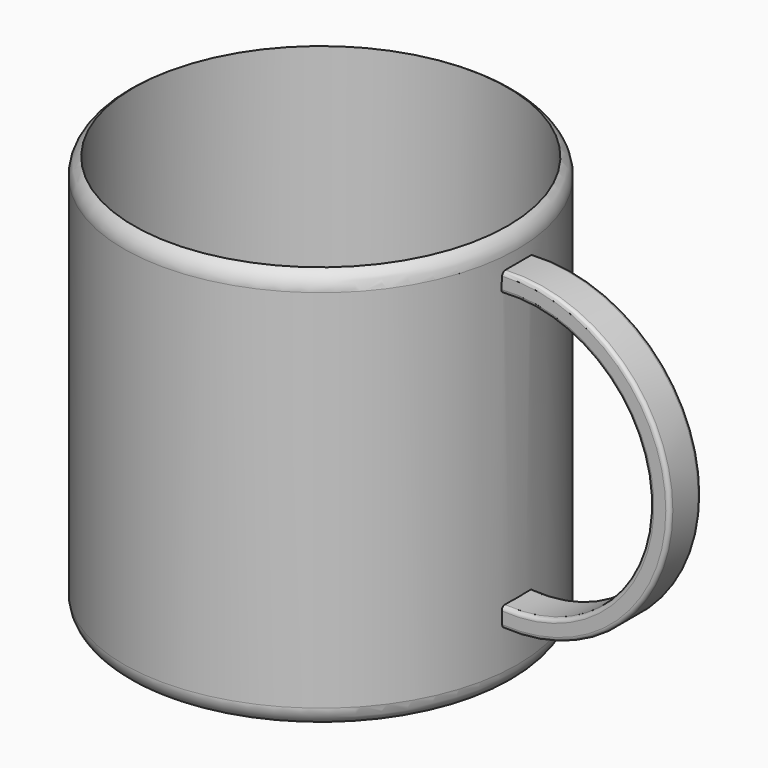
from build123d import *

# Parameters (mm, degrees)
F0_R     = 50
F0_R_2   = 47.5
F1_DEPTH = 101.6
F4_DEPTH = 5
F6_DEPTH = 5
F7_F1_R  = 1
F7_F2_R  = 1
F7_F3_R  = 1
F7_F4_R  = 1


# Not quite as in the source:
# - a fillet or chamfer that OpenCascade refuses, or shapes differently, is made with other operations: its cross-section is extruded or revolved along the edge and cut away or added


with BuildPart() as f1:
    # F0 (on Top) → F1 (new body)
    with BuildSketch(Plane.XY):
        Circle(F0_R)
        Circle(F0_R_2, mode=Mode.SUBTRACT)
    extrude(amount=F1_DEPTH)

    # F2: fillet of radius 5.08 on 1 edges, made by hand

    # F2_s1 → F2_t2 (revolve, cut)
    with BuildSketch(Plane.XZ):
        with BuildLine():
            ThreePointArc((50, 97.2239287026), (49.3309409427, 99.7438493363), (47.5, 101.6))
            Line((47.5, 101.6), (50, 101.6))
            Line((50, 101.6), (50, 97.2239287026))
        make_face()
    revolve(axis=Axis((0, 0, 101.6), (0, 0, 1)), mode=Mode.SUBTRACT)

    # F3: fillet of radius 5.08 on 1 edges, made by hand

    # F3_s1 → F3_t2 (revolve, cut)
    with BuildSketch(Plane.XZ):
        with BuildLine():
            ThreePointArc((50, 4.3760712974), (49.3309409427, 1.8561506637), (47.5, 0))
            Line((47.5, 0), (50, 0))
            Line((50, 0), (50, 4.3760712974))
        make_face()
    revolve(axis=Axis((0, 0, 0), (0, 0, 1)), mode=Mode.SUBTRACT)

    # F0 (on Top) → F4 (join)
    with BuildSketch(Plane.XY):
        Circle(F0_R_2)
    extrude(amount=F4_DEPTH)

    # F5 (on Front) → F6 (join, symmetric)
    with BuildSketch(Plane.XZ):
        with BuildLine():
            Line((49.9294716591, 19.3719161714), (50.0663593411, 14.3504645675))
            ThreePointArc((50.0663593411, 14.3504645675), (92.5802970628, 54.2713878676), (50.0663593411, 94.1923111677))
            Line((50.0663593411, 94.1923111677), (49.7880062733, 89.1598259546))
            ThreePointArc((49.7880062733, 89.1598259546), (87.5802251549, 54.3423353762), (49.9294716591, 19.3719161714))
        make_face()
    extrude(amount=F6_DEPTH, both=True)

    # F7: fillet of radius 1 on 4 edges, made by hand

    # F7_f1
    f7_f1_edges = [f1.edges().sort_by_distance(p)[0] for p in [
        (87.5802251549, -5, 54.3423353762),
    ]]
    fillet(f7_f1_edges, radius=F7_F1_R)

    # F7_f2
    f7_f2_edges = [f1.edges().sort_by_distance(p)[0] for p in [
        (92.5802970628, -5, 54.2713878676),
    ]]
    fillet(f7_f2_edges, radius=F7_F2_R)

    # F7_f3
    f7_f3_edges = [f1.edges().sort_by_distance(p)[0] for p in [
        (92.5802970628, 5, 54.2713878676),
    ]]
    fillet(f7_f3_edges, radius=F7_F3_R)

    # F7_f4
    f7_f4_edges = [f1.edges().sort_by_distance(p)[0] for p in [
        (87.5802251549, 5, 54.3423353762),
    ]]
    fillet(f7_f4_edges, radius=F7_F4_R)


solid = f1.part
